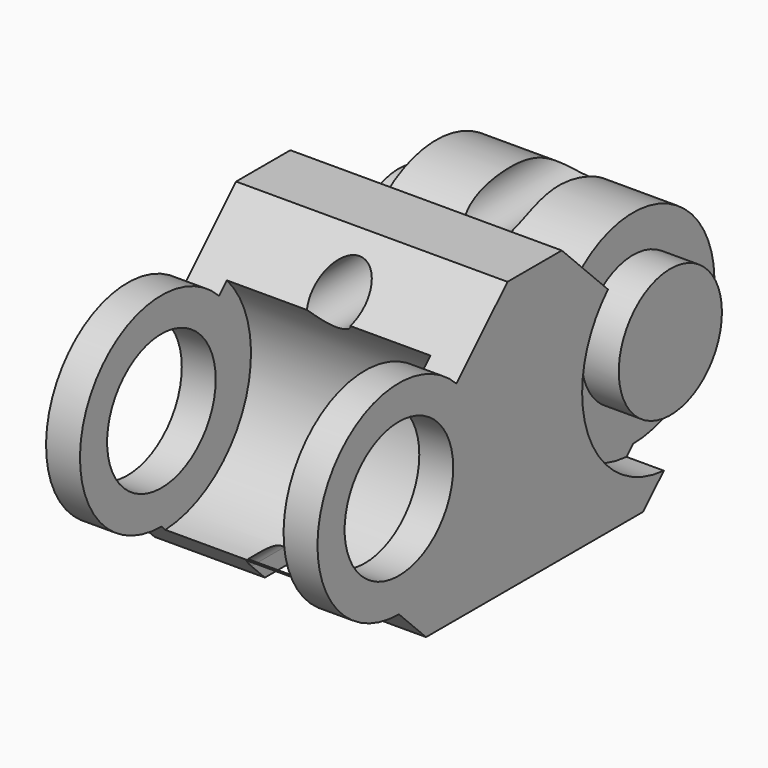
from build123d import *

# Parameters (mm, degrees)
F0_W          = 8
F0_H          = 10
F1_DEPTH      = 8
F2_SIZE       = 4
F4_DEPTH      = 4
F5_DEPTH      = 3
F6_R          = 3.3
F7_DEPTH      = 3
F9_DEPTH      = 1.1
F11_R         = 1.9
F12_DEPTH     = 4
F13_R         = 2
F14_DEPTH     = 12.5
F15_T1_DEPTH  = 13.1433659759
F15_T6_DEPTH  = 13.1433659759
F15_S7_R      = 3
F15_T8_DEPTH  = 8
F16_W         = 1.5
F16_H         = 1.0667801354
F16_H_2       = 8
F16_H_3       = 0.8089432385
F17_DEPTH     = 1
F18_T4_DEPTH  = 11.5268513298
F18_S7_R      = 3.3
F18_T8_DEPTH  = 7
F18_T12_DEPTH = 11.5268513298
F18_S14_R     = 3.3
F18_T15_DEPTH = 7
F19_R         = 0.75
F20_DEPTH     = 25


# Not quite as in the source:
# - a fillet or chamfer that OpenCascade refuses, or shapes differently, is made with other operations: its cross-section is extruded or revolved along the edge and cut away or added


with BuildPart() as f1:
    # F0 (on Top) → F1 (new body)
    with BuildSketch(Plane.XY):
        with Locations((0, 5)):
            Rectangle(F0_W, F0_H)
    extrude(amount=F1_DEPTH)

    # F2
    f2_edges = [f1.edges().sort_by_distance(p)[0] for p in [
        (0, 0, 8),
        (0, 10, 8),
    ]]
    chamfer(f2_edges, length=F2_SIZE)

    # F3 (on Right) → F4 (join, symmetric)
    with BuildSketch(Plane.YZ):
        with BuildLine():
            ThreePointArc((2.1213203436, 6.1213203436), (-2.7716385975, 5.1480502971), (0, 1))
            Line((0, 1), (0, 4))
            Line((0, 4), (2.1213203436, 6.1213203436))
        make_face()
    extrude(amount=F4_DEPTH, both=True)

    # F3 (on Right) → F5 (join, symmetric)
    with BuildSketch(Plane.YZ):
        with BuildLine():
            Line((10, 4), (10, 1))
            ThreePointArc((10, 1), (12.1213203436, 1.8786796564), (13, 4))
            ThreePointArc((13, 4), (11.1480502971, 6.7716385975), (7.8786796564, 6.1213203436))
            Line((7.8786796564, 6.1213203436), (10, 4))
        make_face()
    extrude(amount=F5_DEPTH, both=True)

    # F6 (on Right) → F7 (cut, symmetric)
    with BuildSketch(Plane.YZ):
        with Locations((0, 4.1532493821)):
            Circle(F6_R)
    extrude(amount=F7_DEPTH, both=True, mode=Mode.SUBTRACT)

    # F8 (on face) → F9 (cut)
    with BuildSketch(Plane(origin=(-4, 0, 0), x_dir=(0, -1, 0), z_dir=(-1, 0, 0))):
        with BuildLine():
            Line((-10, 4), (-7.7019029611, 6.2980970389))
            ThreePointArc((-7.7019029611, 6.2980970389), (-13.0026084807, 5.2437211552), (-10, 0.75))
            Line((-10, 0.75), (-10, 4))
        make_face()
        with BuildLine():
            ThreePointArc((-10, 0.75), (-7.7019029611, 1.7019029611), (-6.75, 4))
            ThreePointArc((-6.75, 4), (-6.9973915193, 5.2437211552), (-7.7019029611, 6.2980970389))
            Line((-7.7019029611, 6.2980970389), (-10, 4))
            Line((-10, 4), (-10, 0.75))
        make_face()
    extrude(amount=-F9_DEPTH, mode=Mode.SUBTRACT)

    # F10: F1 across plane


with BuildPart() as f1_1:
    add(f1.part)
    add(f1.part.mirror(Plane.YZ), mode=Mode.INTERSECT)

    # F11 (on Right) → F12 (join, symmetric)
    with BuildSketch(Plane.YZ):
        with Locations((10, 4)):
            Circle(F11_R)
    extrude(amount=F12_DEPTH, both=True)

    # F13 (on Right) → F14 (cut, symmetric)
    with BuildSketch(Plane.YZ):
        with Locations((0, 4)):
            Circle(F13_R)
    extrude(amount=F14_DEPTH, both=True, mode=Mode.SUBTRACT)

    # F15: chamfer of 1 on 2 edges, made by hand

    # F15_s2 → F15_t1 (cut)
    with BuildSketch(Plane.YZ.offset(-6.571682988)):
        Polygon((1, 0), (0, 1), (0, 0), align=None)
    extrude(amount=F15_T1_DEPTH, mode=Mode.SUBTRACT)


with BuildPart() as f15_tool4:
    # F15_s5 → F15_t6 (new body)
    with BuildSketch(Plane.YZ.offset(6.571682988)):
        Polygon((9, 0), (10, 1), (10, 0), align=None)
    extrude(amount=-F15_T6_DEPTH)

    # F15_s7 → F15_t8 (cut, symmetric)
    with BuildSketch(Plane.YZ):
        with Locations((10, 4)):
            Circle(F15_S7_R)
    extrude(amount=F15_T8_DEPTH, both=True, mode=Mode.SUBTRACT)


with BuildPart() as f1_2:
    add(f1_1.part)

    # F15_t3: cut F15_tool4
    add(f15_tool4.part, mode=Mode.SUBTRACT)

    # F16 (on face) → F17 (cut)
    with BuildSketch(Plane(origin=(0, 0, 0), x_dir=(1, 0, 0), z_dir=(0, 0, -1))):
        with Locations((0, -9.5333900677)):
            Rectangle(F16_W, F16_H)
        with Locations((0, -5)):
            Rectangle(F16_W, F16_H_2)
        with Locations((0, -0.5955283808)):
            Rectangle(F16_W, F16_H_3)
    extrude(amount=-F17_DEPTH, mode=Mode.SUBTRACT)

    # F18: fillet of radius 0.5 on 2 edges, made by hand


with BuildPart() as f18_tool2:
    # F18_s3 → F18_t4 (new body)
    with BuildSketch(Plane.XZ.offset(0.2768513298)):
        with BuildLine():
            ThreePointArc((-0.75, 0.5), (-0.6035533906, 0.8535533906), (-0.25, 1))
            Line((-0.25, 1), (-0.75, 1))
            Line((-0.75, 1), (-0.75, 0.5))
        make_face()
    extrude(amount=-F18_T4_DEPTH)

    split(bisect_by=Plane(origin=(0, 0.5, 0.5), x_dir=(1, 0, 0), z_dir=(0, 0.7071067812, 0.7071067812)), keep=Keep.TOP)

    split(bisect_by=Plane(origin=(0, 4.5, -4.5), x_dir=(1, 0, 0), z_dir=(0, -0.7071067812, 0.7071067812)), keep=Keep.TOP)

    # F18_s7 → F18_t8 (cut, symmetric)
    with BuildSketch(Plane.YZ.offset(-0.5)):
        with Locations((0, 4.1532493821)):
            Circle(F18_S7_R)
    extrude(amount=F18_T8_DEPTH, both=True, mode=Mode.SUBTRACT)


with BuildPart() as f1_3:
    add(f1_2.part)

    # F18_t1: union F18_tool2
    add(f18_tool2.part)


with BuildPart() as f18_tool10:
    # F18_s11 → F18_t12 (new body)
    with BuildSketch(Plane.XZ.offset(-11.25)):
        with BuildLine():
            ThreePointArc((0.75, 0.5), (0.6035533906, 0.8535533906), (0.25, 1))
            Line((0.25, 1), (0.75, 1))
            Line((0.75, 1), (0.75, 0.5))
        make_face()
    extrude(amount=F18_T12_DEPTH)

    split(bisect_by=Plane(origin=(0, 0.5, 0.5), x_dir=(1, 0, 0), z_dir=(0, 0.7071067812, 0.7071067812)), keep=Keep.TOP)

    # F18_s14 → F18_t15 (cut, symmetric)
    with BuildSketch(Plane.YZ.offset(0.5)):
        with Locations((0, 4.1532493821)):
            Circle(F18_S14_R)
    extrude(amount=F18_T15_DEPTH, both=True, mode=Mode.SUBTRACT)

    split(bisect_by=Plane(origin=(0, 4.5, -4.5), x_dir=(1, 0, 0), z_dir=(0, -0.7071067812, 0.7071067812)), keep=Keep.TOP)


with BuildPart() as f1_4:
    add(f1_3.part)

    # F18_t9: union F18_tool10
    add(f18_tool10.part)

    # F19 (on Front) → F20 (cut)
    with BuildSketch(Plane.XZ):
        with Locations((0, 6.8)):
            Circle(F19_R)
    extrude(amount=-F20_DEPTH, mode=Mode.SUBTRACT)


solid = f1_4.part
